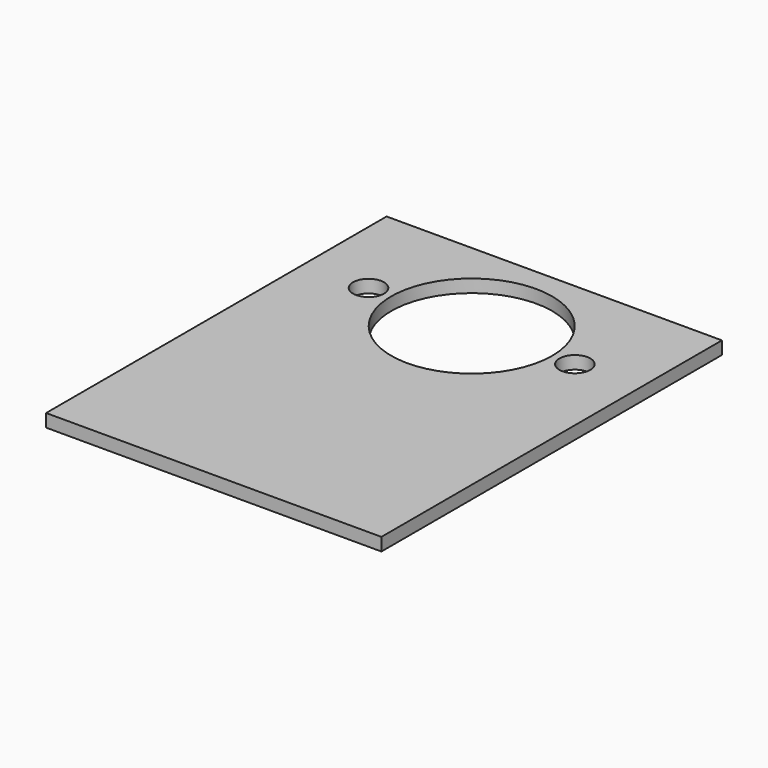
from build123d import *

# Parameters (mm, degrees)
F0_W     = 82.55
F0_H     = 104.775
F1_DEPTH = 3.175
F2_R     = 19.812
F2_R_2   = 3.81
F3_DEPTH = 25.4


# Not quite as in the source:
# - a feature names something its author has since deleted; it is built from what else it names


with BuildPart() as f1:
    # F0 (on Top) → F1 (new body)
    with BuildSketch(Plane.XY):
        with Locations((0, -26.9875)):
            Rectangle(F0_W, F0_H)
    extrude(amount=F1_DEPTH)

    # F2 (on face) → F3 (cut)
    with BuildSketch(Plane.XY.offset(3.175)):
        Circle(F2_R)
        with Locations((-25.4, 0)):
            Circle(F2_R_2)
        with Locations((25.4, 0)):
            Circle(F2_R_2)
    extrude(amount=-F3_DEPTH, mode=Mode.SUBTRACT)


solid = f1.part
